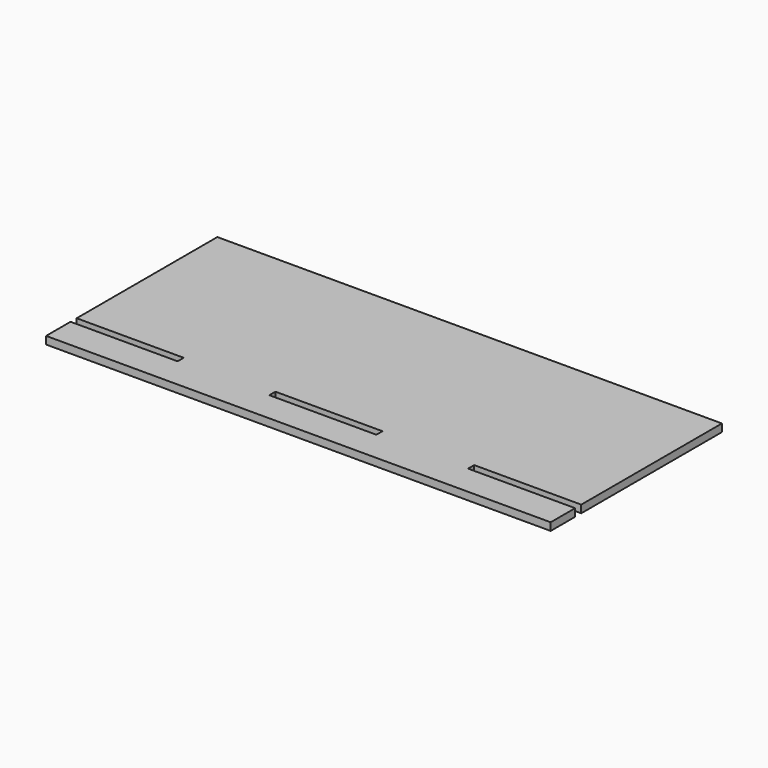
from build123d import *

# Parameters (mm, degrees)
F0_W     = 209.55
F0_H     = 88.9
F1_DEPTH = 3.175
F2_W     = 44.45
F2_H     = 3.175
F3_DEPTH = 25.4


# Not quite as in the source:
# - a length typed as a fraction of an inch, garbled in the dataset ("3 / 203.2 mm" for 3/8 in), is restored


with BuildPart() as f1:
    # F0 (on Top) → F1 (new body)
    with BuildSketch(Plane.XY):
        Rectangle(F0_W, F0_H)
    extrude(amount=F1_DEPTH)

    # F2 (on face) → F3 (cut)
    with BuildSketch(Plane.XY.offset(3.175)):
        with Locations((-82.55, -30.1625)):
            Rectangle(F2_W, F2_H)
        with Locations((82.55, -30.1625)):
            Rectangle(F2_W, F2_H)
        with Locations((0, -30.1625)):
            Rectangle(F2_W, F2_H)
    extrude(amount=-F3_DEPTH, mode=Mode.SUBTRACT)


solid = f1.part
